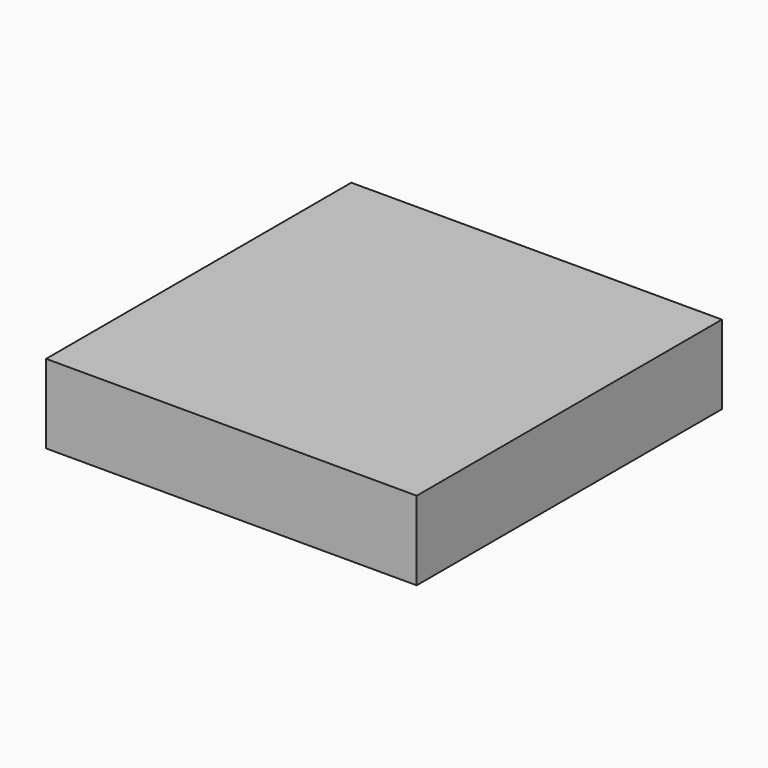
from build123d import *

# Parameters (mm, degrees)
F0_W     = 151.3053178787
F0_H     = 155.7376980782
F2_DEPTH = 32.2132073343


# Not quite as in the source:
# - the program builds the solid bodies; features that only make, move or delete a surface that nothing else refers to are left out


with BuildPart() as f2:
    # F0 (on Top) → F2 (new body)
    with BuildSketch(Plane.XY):
        Rectangle(F0_W, F0_H)
    extrude(amount=F2_DEPTH)


solid = f2.part
